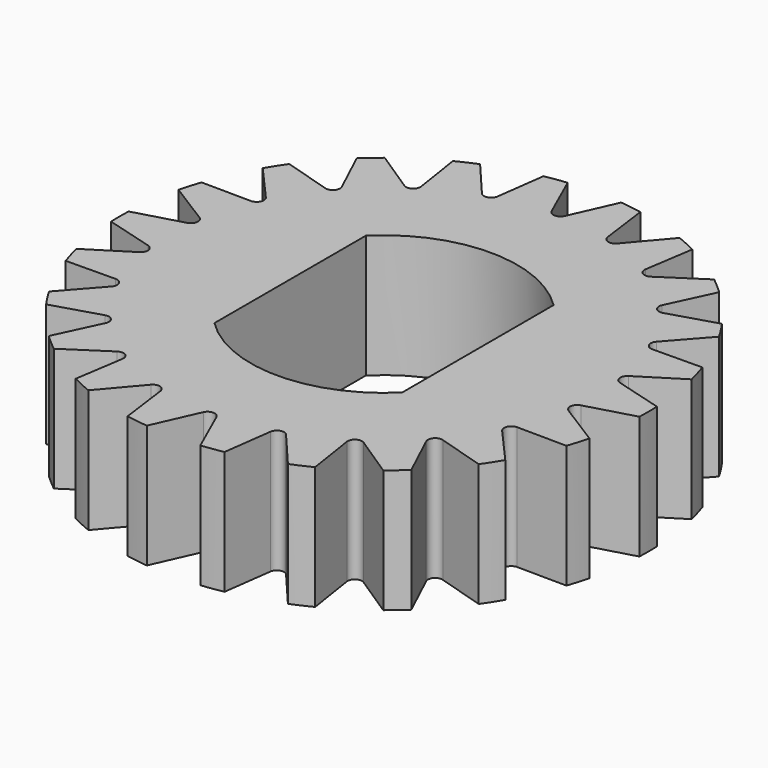
from build123d import *

# Parameters (mm, degrees)
F0_R            = 10.909800859
F1_DEPTH        = 5.08
F3_DEPTH        = 5.08
F3_COPIES_COUNT = 22


# Not quite as in the source:
# - a pattern or mirror of a feature is missing from the dataset's text; its kind, count and spacing are read off the source's solid


with BuildPart() as f1:
    # F0 (on Top) → F1 (new body)
    with BuildSketch(Plane.XY):
        Circle(F0_R)
        with BuildLine():
            ThreePointArc((3.8749986, -3.9031251389), (0, -5.5), (-3.8749986, -3.9031251389))
            Line((-3.8749986, -3.9031251389), (-3.8749986, 3.9031251389))
            ThreePointArc((-3.8749986, 3.9031251389), (0, 5.5), (3.8749986, 3.9031251389))
            Line((3.8749986, 3.9031251389), (3.8749986, -3.9031251389))
        make_face(mode=Mode.SUBTRACT)
    extrude(amount=F1_DEPTH)

    # F2 (on face) → F3 (cut, through all)
    with BuildSketch(Plane.XY.offset(5.08)):
        with BuildLine():
            Line((0.2718847261, 8.9821943232), (1.1039126824, 10.8538072386))
            ThreePointArc((1.1039126824, 10.8538072386), (0, 10.909800859), (-1.1039126824, 10.8538072386))
            Line((-1.1039126824, 10.8538072386), (-0.2718847261, 8.9821943232))
            ThreePointArc((-0.2718847261, 8.9821943232), (0, 8.8055210085), (0.2718847261, 8.9821943232))
        make_face()
    f3 = extrude(amount=-F3_DEPTH, mode=Mode.SUBTRACT)

    # F3_copies: F3 ×22 about axis
    f3_copies_axis = Axis((0, 0, 0), (0, 0, 1))
    for i in range(1, F3_COPIES_COUNT):
        add(f3.rotate(f3_copies_axis, i * 360 / F3_COPIES_COUNT), mode=Mode.SUBTRACT)


solid = f1.part
